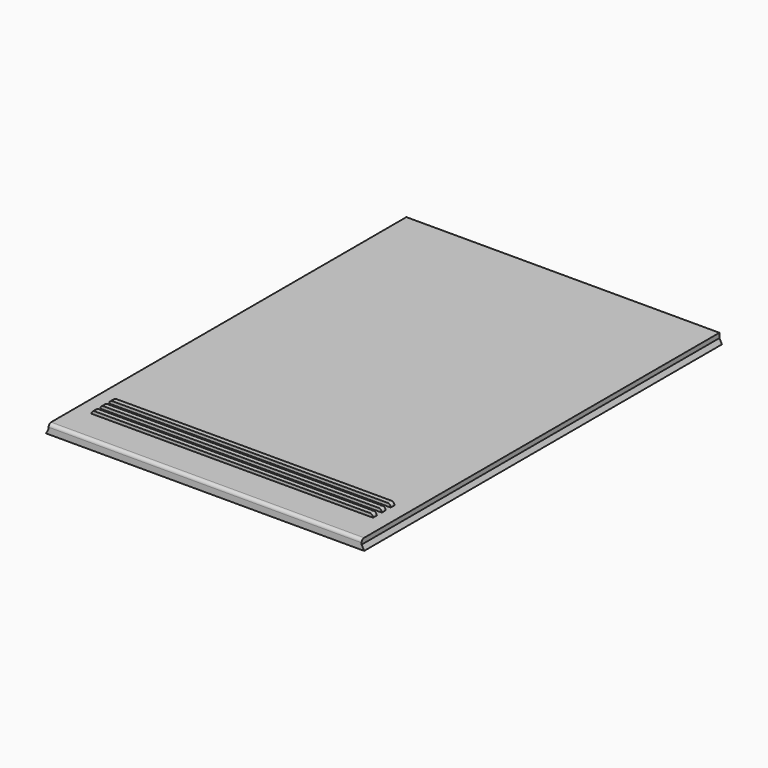
from build123d import *

# Parameters (mm, degrees)
F0_W     = 49.7
F0_H     = 1.5
F1_DEPTH = 142
F2_W     = 44.6868650615
F2_H     = 1.5
F3_DEPTH = 1
F4_R     = 0.99999


# Not quite as in the source:
# - a fillet or chamfer is up to 0.001 mm smaller than in the source, because OpenCascade refuses the exact size


with BuildPart() as f1:
    # F0 (on Front) → F1 (new body)
    with BuildSketch(Plane.XZ):
        with Locations((24.85, -0.75)):
            Rectangle(F0_W, F0_H)
        with Locations((-24.85, -0.75)):
            Rectangle(F0_W, F0_H)
        Polygon((49.7, -1.5), (0, -1.5), (0, -3), (50.5, -3), align=None)
        Polygon((0, -3), (0, -1.5), (-49.7, -1.5), (-50.5, -3), align=None)
    extrude(amount=F1_DEPTH)

    # F2 (on face) → F3 (join)
    with BuildSketch(Plane.XY):
        with Locations((-22.3434325308, -130.4639992552)):
            Rectangle(F2_W, F2_H)
        with Locations((22.3434325308, -130.4639992552)):
            Rectangle(F2_W, F2_H)
        with Locations((-22.3434325308, -126.9639992552)):
            Rectangle(F2_W, F2_H)
        with Locations((22.3434325308, -126.9639992552)):
            Rectangle(F2_W, F2_H)
        with Locations((-22.3434325308, -123.4639992552)):
            Rectangle(F2_W, F2_H)
        with Locations((22.3434325308, -123.4639992552)):
            Rectangle(F2_W, F2_H)
    extrude(amount=F3_DEPTH)

    # F4 (radius 1 in the source; OpenCascade refuses exactly that, so slightly less here)
    f4_edges = [f1.edges().sort_by_distance(p)[0] for p in [
        (-44.686865, -123.463999, 1),
        (-44.686865, -126.963999, 1),
        (-44.686865, -130.463999, 1),
        (44.686865, -123.463999, 1),
        (44.686865, -126.963999, 1),
        (44.686865, -130.463999, 1),
        (0, -142, 0),
    ]]
    fillet(f4_edges, radius=F4_R)


solid = f1.part
